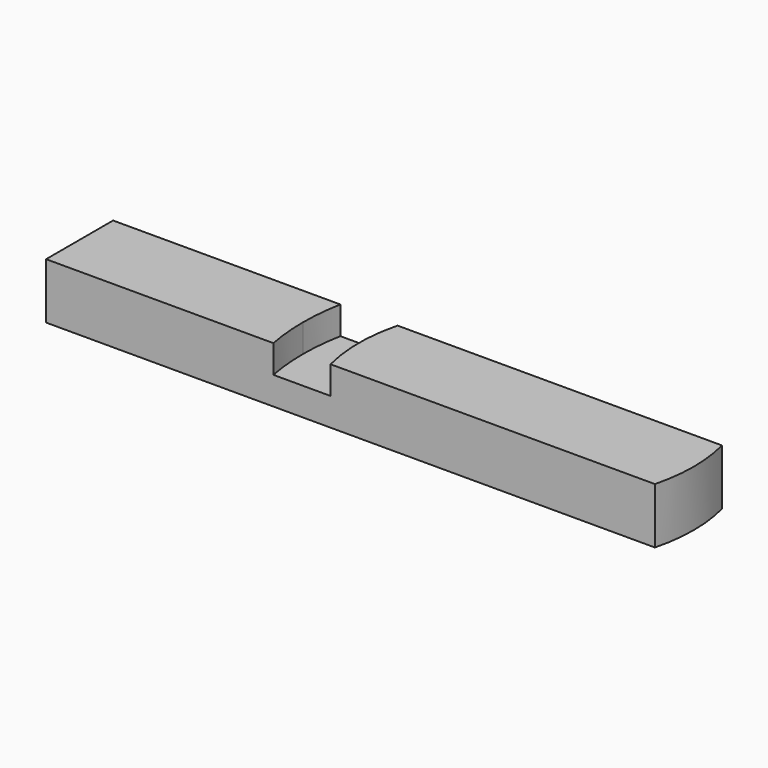
from build123d import *

# Parameters (mm, degrees)
F0_W     = 36.8901663726
F0_H     = 9.525
F1_DEPTH = 3.175
F2_DEPTH = 3.175


with BuildPart() as f1:
    # F0 (on Top) → F1 (new body)
    with BuildSketch(Plane.XY):
        with BuildLine():
            ThreePointArc((18.4450831863, -4.7625), (18.8981657139, -2.4003817718), (19.05, 0))
            ThreePointArc((19.05, 0), (18.8981657139, 2.4003817718), (18.4450831863, 4.7625))
            Line((18.4450831863, 4.7625), (18.4450831863, -4.7625))
        make_face()
        Rectangle(F0_W, F0_H)
        with BuildLine():
            Line((-18.4450831863, -4.7625), (-18.4450831863, 4.7625))
            ThreePointArc((-18.4450831863, 4.7625), (-19.05, 0), (-18.4450831863, -4.7625))
        make_face()
    extrude(amount=F1_DEPTH)



with BuildPart() as f1b:
    # F0 (on Top) → F1, piece 2 (new body)
    with BuildSketch(Plane.XY):
        with BuildLine():
            ThreePointArc((-25.4, 0), (-25.2871294453, 2.3918788461), (-24.9495209122, 4.7625))
            Line((-24.9495209122, 4.7625), (-25.4, 4.7625))
            Line((-25.4, 4.7625), (-25.4, 0))
        make_face()
        with BuildLine():
            Line((-25.4, -4.7625), (-24.9495209122, -4.7625))
            ThreePointArc((-24.9495209122, -4.7625), (-25.2871294453, -2.3918788461), (-25.4, 0))
            Line((-25.4, 0), (-25.4, -4.7625))
        make_face()
        Polygon((-25.4, 0), (-25.4, 4.7625), (-50.8, 4.7625), (-50.8, -4.7625), (-25.4, -4.7625), align=None)
    extrude(amount=F1_DEPTH)


with BuildPart() as f1_1:
    add(f1.part)

    add(f1b.part)  # F2 merges F1b
    # F0 (on Top) → F2 (join)
    with BuildSketch(Plane.XY):
        with BuildLine():
            ThreePointArc((18.4450831863, -4.7625), (18.8981657139, -2.4003817718), (19.05, 0))
            ThreePointArc((19.05, 0), (18.8981657139, 2.4003817718), (18.4450831863, 4.7625))
            Line((18.4450831863, 4.7625), (18.4450831863, -4.7625))
        make_face()
        Rectangle(F0_W, F0_H)
        with BuildLine():
            Line((-18.4450831863, -4.7625), (-18.4450831863, 4.7625))
            ThreePointArc((-18.4450831863, 4.7625), (-19.05, 0), (-18.4450831863, -4.7625))
        make_face()
        with BuildLine():
            ThreePointArc((-18.4450831863, -4.7625), (-19.05, 0), (-18.4450831863, 4.7625))
            Line((-18.4450831863, 4.7625), (-24.9495209122, 4.7625))
            ThreePointArc((-24.9495209122, 4.7625), (-25.2871294453, 2.3918788461), (-25.4, 0))
            ThreePointArc((-25.4, 0), (-25.2871294453, -2.3918788461), (-24.9495209122, -4.7625))
            Line((-24.9495209122, -4.7625), (-18.4450831863, -4.7625))
        make_face()
        with BuildLine():
            ThreePointArc((-25.4, 0), (-25.2871294453, 2.3918788461), (-24.9495209122, 4.7625))
            Line((-24.9495209122, 4.7625), (-25.4, 4.7625))
            Line((-25.4, 4.7625), (-25.4, 0))
        make_face()
        with BuildLine():
            Line((-25.4, -4.7625), (-24.9495209122, -4.7625))
            ThreePointArc((-24.9495209122, -4.7625), (-25.2871294453, -2.3918788461), (-25.4, 0))
            Line((-25.4, 0), (-25.4, -4.7625))
        make_face()
        Polygon((-25.4, 0), (-25.4, 4.7625), (-50.8, 4.7625), (-50.8, -4.7625), (-25.4, -4.7625), align=None)
    extrude(amount=-F2_DEPTH)


solid = f1_1.part
